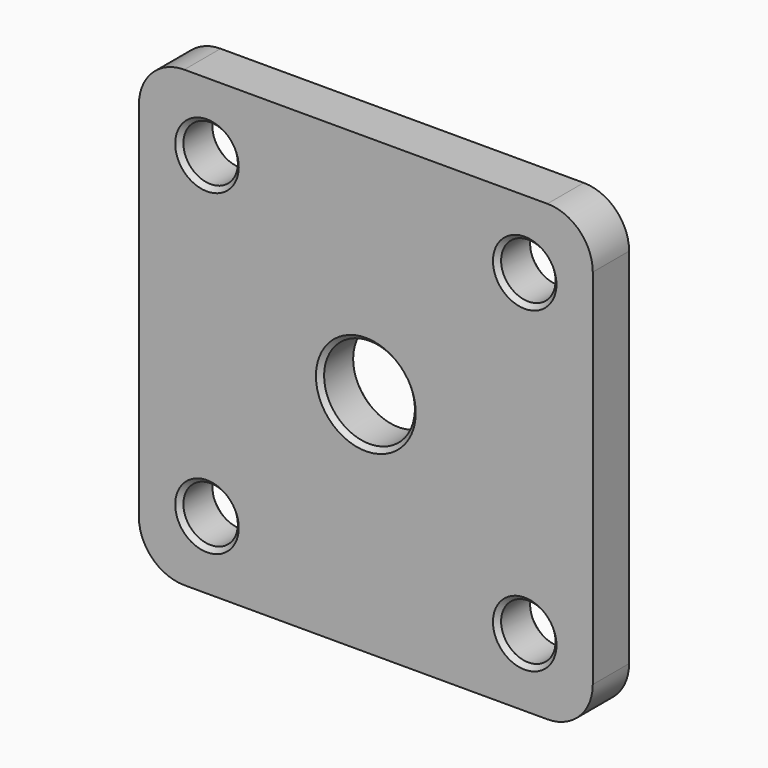
from build123d import *

# Parameters (mm, degrees)
F0_W     = 100
F0_H     = 100
F0_R     = 6
F1_DEPTH = 10
F3_D     = 20
F4_R     = 10
F5_SIZE  = 1


with BuildPart() as f1:
    # F0 (on Front) → F1 (new body)
    with BuildSketch(Plane.XZ):
        Rectangle(F0_W, F0_H)
        with Locations((-35, -35)):
            Circle(F0_R, mode=Mode.SUBTRACT)
        with Locations((35, -35)):
            Circle(F0_R, mode=Mode.SUBTRACT)
        with Locations((-35, 35)):
            Circle(F0_R, mode=Mode.SUBTRACT)
        with Locations((35, 35)):
            Circle(F0_R, mode=Mode.SUBTRACT)
    extrude(amount=F1_DEPTH)

    # F3 (through all)
    with Locations(Plane.XZ.offset(10)):
        with Locations((0, 0)):
            Hole(F3_D / 2)

    # F4
    f4_edges = [f1.edges().sort_by_distance(p)[0] for p in [
        (-50, -5, -50),
        (50, -5, -50),
        (50, -5, 50),
        (-50, -5, 50),
    ]]
    fillet(f4_edges, radius=F4_R)

    # F5
    f5_edges = [f1.edges().sort_by_distance(p)[0] for p in [
        (-41, -10, 35),
        (29, -10, 35),
        (29, -10, -35),
        (-41, -10, -35),
        (-41, 0, 35),
        (-41, 0, -35),
        (29, 0, -35),
        (29, 0, 35),
        (-10, 0, 0),
        (-10, -10, 0),
    ]]
    chamfer(f5_edges, length=F5_SIZE)


solid = f1.part
